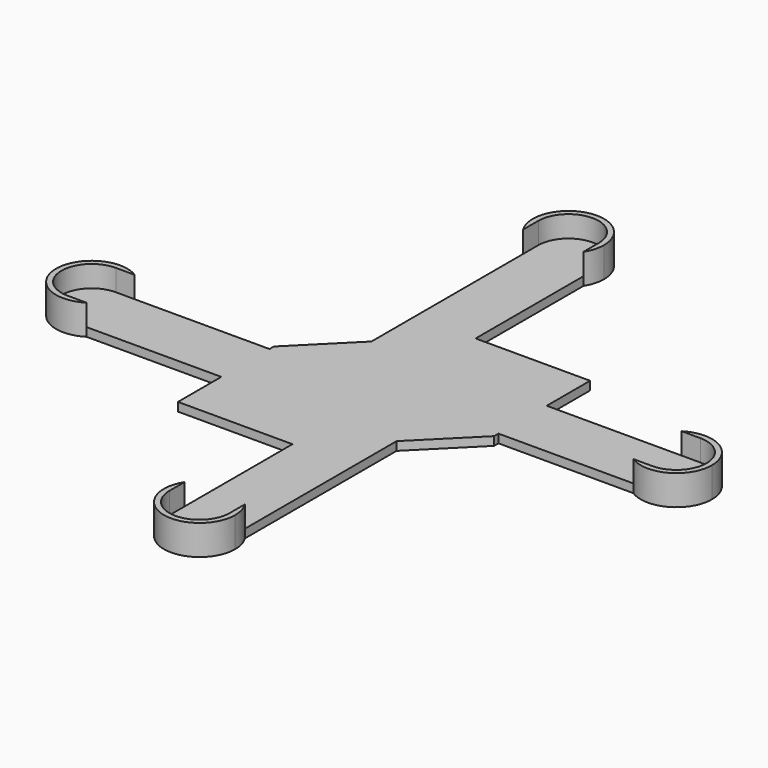
from build123d import *

# Parameters (mm, degrees)
F1_DEPTH    = 4
F2_DEPTH    = 14
F3_W        = 53.352586925
F3_H        = 25.252586925
F4_DEPTH    = 4
F3_W_2      = 25.252586925
F3_H_2      = 53.352586925
F5_DEPTH    = 4
F6_T4_DEPTH = 265.2829915773
F6_T9_DEPTH = 265.2829915773


# Not quite as in the source:
# - a fillet or chamfer that OpenCascade refuses, or shapes differently, is made with other operations: its cross-section is extruded or revolved along the edge and cut away or added


with BuildPart() as f1:
    # F0 (on Top) → F1 (new body)
    with BuildSketch(Plane.XY):
        with BuildLine():
            ThreePointArc((0, 125), (-14.05, 139.05), (-28.1, 125))
            Line((-28.1, 125), (0, 125))
        make_face()
        with BuildLine():
            Line((0, 125), (-28.1, 125))
            ThreePointArc((-28.1, 125), (-14.05, 110.95), (0, 125))
        make_face()
        with BuildLine():
            Line((-28.1, 125), (-28.1, 116.1781181146))
            ThreePointArc((-28.1, 116.1781181146), (-14.05, 108.41), (0, 116.1781181146))
            Line((0, 116.1781181146), (0, 125))
            ThreePointArc((0, 125), (-14.05, 110.95), (-28.1, 125))
        make_face()
        with BuildLine():
            Line((-28.1, 0), (0, 0))
            Line((0, 0), (0, 28.1))
            Line((0, 28.1), (0, 116.1781181146))
            ThreePointArc((0, 116.1781181146), (-14.05, 108.41), (-28.1, 116.1781181146))
            Line((-28.1, 116.1781181146), (-28.1, 0))
        make_face()
        with BuildLine():
            Line((0, 28.1), (0, 0))
            Line((0, 0), (28.1, 0))
            Line((28.1, 0), (116.1781181146, 0))
            ThreePointArc((116.1781181146, 0), (108.41, 14.05), (116.1781181146, 28.1))
            Line((116.1781181146, 28.1), (0, 28.1))
        make_face()
        with BuildLine():
            ThreePointArc((139.05, 14.05), (134.9348502757, 23.9848502757), (125, 28.1))
            Line((125, 28.1), (125, 0))
            ThreePointArc((125, 0), (134.9348502757, 4.1151497243), (139.05, 14.05))
        make_face()
        with BuildLine():
            Line((125, 0), (125, 28.1))
            ThreePointArc((125, 28.1), (110.95, 14.05), (125, 0))
        make_face()
        with BuildLine():
            Line((28.1, 0), (0, 0))
            Line((0, 0), (0, -28.1))
            Line((0, -28.1), (0, -116.1781181146))
            ThreePointArc((0, -116.1781181146), (14.05, -108.41), (28.1, -116.1781181146))
            Line((28.1, -116.1781181146), (28.1, 0))
        make_face()
        with BuildLine():
            Line((28.1, -125), (0, -125))
            ThreePointArc((0, -125), (14.05, -139.05), (28.1, -125))
        make_face()
        with BuildLine():
            ThreePointArc((28.1, -125), (14.05, -110.95), (0, -125))
            Line((0, -125), (28.1, -125))
        make_face()
        with BuildLine():
            ThreePointArc((28.1, -116.1781181146), (14.05, -108.41), (0, -116.1781181146))
            Line((0, -116.1781181146), (0, -125))
            ThreePointArc((0, -125), (14.05, -110.95), (28.1, -125))
            Line((28.1, -125), (28.1, -116.1781181146))
        make_face()
        with BuildLine():
            Line((-125, -28.1), (-125, 0))
            ThreePointArc((-125, 0), (-139.05, -14.05), (-125, -28.1))
        make_face()
        with BuildLine():
            ThreePointArc((-110.95, -14.05), (-115.0651497243, -4.1151497243), (-125, 0))
            Line((-125, 0), (-125, -28.1))
            ThreePointArc((-125, -28.1), (-115.0651497243, -23.9848502757), (-110.95, -14.05))
        make_face()
        with BuildLine():
            ThreePointArc((-108.41, -14.05), (-110.4813375189, -6.0227626321), (-116.1781181146, 0))
            Line((-116.1781181146, 0), (-125, 0))
            ThreePointArc((-125, 0), (-115.0651497243, -4.1151497243), (-110.95, -14.05))
            ThreePointArc((-110.95, -14.05), (-115.0651497243, -23.9848502757), (-125, -28.1))
            Line((-125, -28.1), (-116.1781181146, -28.1))
            ThreePointArc((-116.1781181146, -28.1), (-110.4813375189, -22.0772373679), (-108.41, -14.05))
        make_face()
        with BuildLine():
            Line((0, -28.1), (0, 0))
            Line((0, 0), (-28.1, 0))
            Line((-28.1, 0), (-116.1781181146, 0))
            ThreePointArc((-116.1781181146, 0), (-110.4813375189, -6.0227626321), (-108.41, -14.05))
            ThreePointArc((-108.41, -14.05), (-110.4813375189, -22.0772373679), (-116.1781181146, -28.1))
            Line((-116.1781181146, -28.1), (0, -28.1))
        make_face()
        with BuildLine():
            Line((125, 28.1), (116.1781181146, 28.1))
            ThreePointArc((116.1781181146, 28.1), (108.41, 14.05), (116.1781181146, 0))
            Line((116.1781181146, 0), (125, 0))
            ThreePointArc((125, 0), (110.95, 14.05), (125, 28.1))
        make_face()
    extrude(amount=F1_DEPTH)

    # F0 (on Top) → F2 (join)
    with BuildSketch(Plane.XY):
        with BuildLine():
            ThreePointArc((2.54, 125), (-18.6401307171, 140.9423586712), (-28.1, 116.1781181146))
            Line((-28.1, 116.1781181146), (-28.1, 125))
            ThreePointArc((-28.1, 125), (-14.05, 139.05), (0, 125))
            Line((0, 125), (0, 116.1781181146))
            ThreePointArc((0, 116.1781181146), (1.8923586712, 120.4098692829), (2.54, 125))
        make_face()
        with BuildLine():
            ThreePointArc((141.59, 14.05), (133.0272373679, 28.5686624811), (116.1781181146, 28.1))
            Line((116.1781181146, 28.1), (125, 28.1))
            ThreePointArc((125, 28.1), (134.9348502757, 23.9848502757), (139.05, 14.05))
            ThreePointArc((139.05, 14.05), (134.9348502757, 4.1151497243), (125, 0))
            Line((125, 0), (116.1781181146, 0))
            ThreePointArc((116.1781181146, 0), (133.0272373679, -0.4686624811), (141.59, 14.05))
        make_face()
        with BuildLine():
            Line((0, -125), (0, -116.1781181146))
            ThreePointArc((0, -116.1781181146), (9.4598692829, -140.9423586712), (30.64, -125))
            ThreePointArc((30.64, -125), (29.9923586712, -120.4098692829), (28.1, -116.1781181146))
            Line((28.1, -116.1781181146), (28.1, -125))
            ThreePointArc((28.1, -125), (14.05, -139.05), (0, -125))
        make_face()
        with BuildLine():
            Line((-125, 0), (-116.1781181146, 0))
            ThreePointArc((-116.1781181146, 0), (-141.59, -14.05), (-116.1781181146, -28.1))
            Line((-116.1781181146, -28.1), (-125, -28.1))
            ThreePointArc((-125, -28.1), (-139.05, -14.05), (-125, 0))
        make_face()
    extrude(amount=F2_DEPTH)

    # F3 (on face) → F4 (join)
    with BuildSketch(Plane.XY.offset(4)):
        with Locations((26.6762934625, 40.7262934625)):
            Rectangle(F3_W, F3_H)
    extrude(amount=-F4_DEPTH)

    # F3 (on face) → F5 (join)
    with BuildSketch(Plane.XY.offset(4)):
        with Locations((40.7262934625, -26.6762934625)):
            Rectangle(F3_W_2, F3_H_2)
        with Locations((-26.6762934625, -40.7262934625)):
            Rectangle(F3_W, F3_H)
        with Locations((-40.7262934625, 26.6762934625)):
            Rectangle(F3_W_2, F3_H_2)
    extrude(amount=-F5_DEPTH)

    # F6: chamfer of 50.8 on 2 edges, made by hand


with BuildPart() as f6_tool2:
    # F6_s3 → F6_t4 (new body)
    with BuildSketch(Plane.XY.offset(134.6414957887)):
        Polygon((2.552586925, -53.352586925), (53.352586925, -2.552586925), (53.352586925, -53.352586925), align=None)
    extrude(amount=-F6_T4_DEPTH)

    split(bisect_by=Plane.YZ.offset(28.1), keep=Keep.TOP)


with BuildPart() as f1_1:
    add(f1.part)

    # F6_t1: cut F6_tool2
    add(f6_tool2.part, mode=Mode.SUBTRACT)


with BuildPart() as f6_tool7:
    # F6_s8 → F6_t9 (new body)
    with BuildSketch(Plane.XY.offset(134.6414957887)):
        Polygon((-2.552586925, 53.352586925), (-53.352586925, 2.552586925), (-53.352586925, 53.352586925), align=None)
    extrude(amount=-F6_T9_DEPTH)

    split(bisect_by=Plane.YZ.offset(-28.1), keep=Keep.BOTTOM)


with BuildPart() as f1_2:
    add(f1_1.part)

    # F6_t6: cut F6_tool7
    add(f6_tool7.part, mode=Mode.SUBTRACT)


solid = f1_2.part
